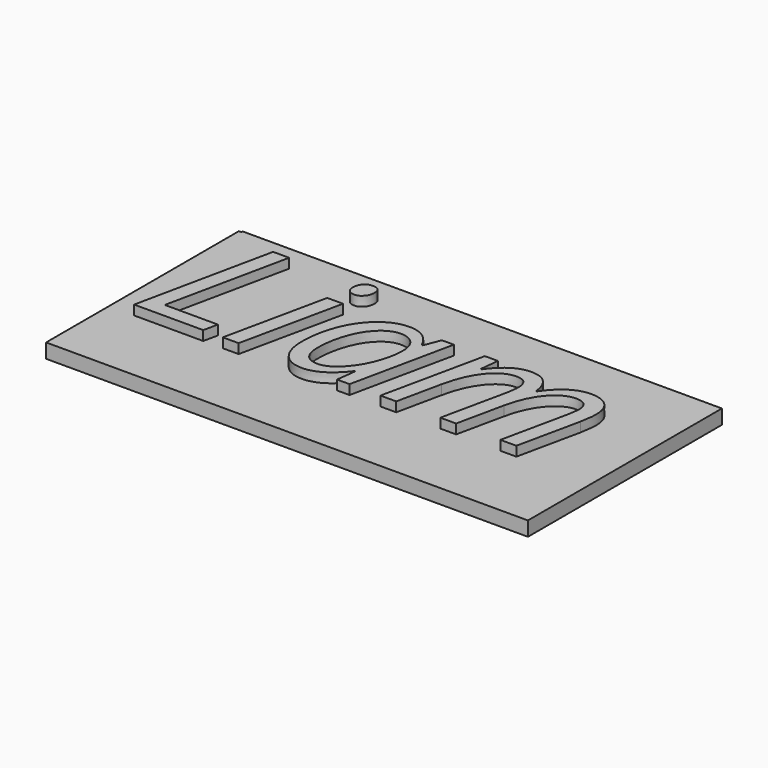
from build123d import *

# Parameters (mm, degrees)
F0_W         = 0.5007544532
F0_H         = 50.1099526882
F0_W_2       = 99.7296562418
F0_H_2       = 0.3306381404
F1_DEPTH     = 3
F2_TEXT_SIZE = 40.0360621926
F3_DEPTH     = 2


# Not quite as in the source:
# - Text() gives the source's letters only with a copy of the font that has no kerning and outlines rounded to 1/6400 em; it was checked with that copy


with BuildPart() as f1:
    # F0 (on Top) → F1 (new body)
    with BuildSketch(Plane.XY):
        with Locations((0.2503772266, 25.0549763441)):
            Rectangle(F0_W, F0_H)
        with Locations((50.3655825742, 25.0549763441)):
            Rectangle(F0_W_2, F0_H)
        with Locations((50.3655825742, 50.2752717584)):
            Rectangle(F0_W_2, F0_H_2)
    extrude(amount=F1_DEPTH)

    # F2 (on face) → F3 (join)
    with BuildSketch(Plane.XY.offset(3)):
        with Locations((3.5689563956, 16.3345634937)):
            Text('Liam', F2_TEXT_SIZE, font='Open Sans', font_style=FontStyle.ITALIC, text_align=(TextAlign.LEFT, TextAlign.BOTTOM))
    extrude(amount=F3_DEPTH)


solid = f1.part
